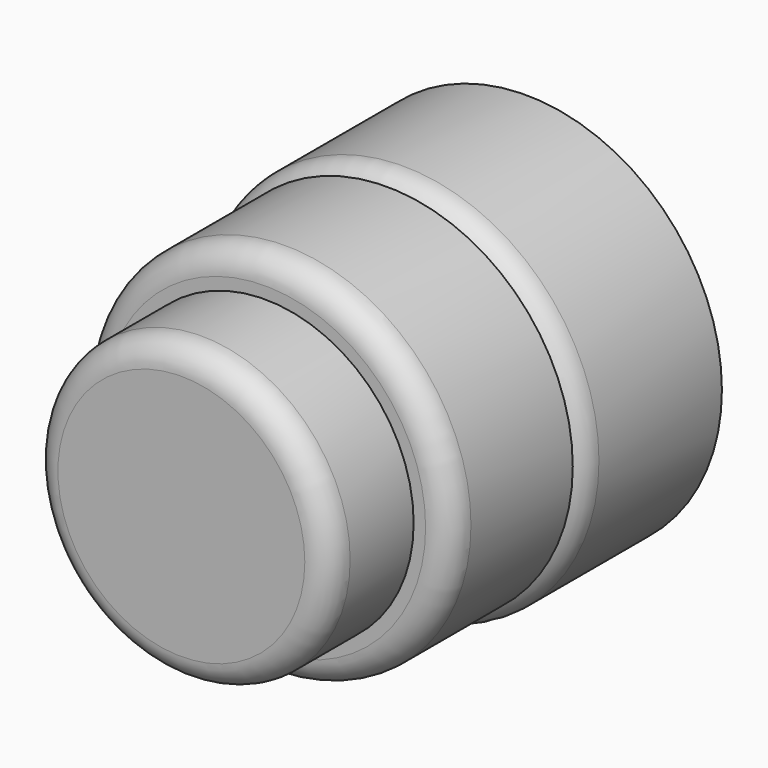
from build123d import *

# Parameters (mm, degrees)
F0_R     = 39.497
F1_DEPTH = 91.186
F2_R     = 39.497
F2_R_2   = 37.465
F3_DEPTH = 56.134
F4_R     = 37.465
F4_R_2   = 32.893
F5_DEPTH = 25.4
F6_R     = 29.972
F7_DEPTH = 21.082
F9_DEPTH = 17.78


# Not quite as in the source:
# - a fillet or chamfer that OpenCascade refuses, or shapes differently, is made with other operations: its cross-section is extruded or revolved along the edge and cut away or added


with BuildPart() as f1:
    # F0 (on Front) → F1 (new body)
    with BuildSketch(Plane.XZ):
        Circle(F0_R)
    extrude(amount=F1_DEPTH)

    # F2 (on face) → F3 (cut)
    with BuildSketch(Plane.XZ.offset(91.186)):
        Circle(F2_R)
        Circle(F2_R_2, mode=Mode.SUBTRACT)
    extrude(amount=-F3_DEPTH, mode=Mode.SUBTRACT)

    # F4 (on face) → F5 (cut)
    with BuildSketch(Plane.XZ.offset(91.186)):
        Circle(F4_R)
        Circle(F4_R_2, mode=Mode.SUBTRACT)
        Circle(F4_R_2)
    extrude(amount=-F5_DEPTH, mode=Mode.SUBTRACT)

    # F6 (on face) → F7 (join)
    with BuildSketch(Plane.XZ.offset(65.786)):
        Circle(F6_R)
    extrude(amount=F7_DEPTH)

    # F8 (on face) → F9 (cut)
    with BuildSketch(Plane(origin=(0, 0, 0), x_dir=(-1, 0, 0), z_dir=(0, 1, 0))):
        with BuildLine():
            ThreePointArc((0, 23.3172), (1.113551759, 23.778448241), (1.5748, 24.892))
            ThreePointArc((1.5748, 24.892), (1.113551759, 26.005551759), (0, 26.4668))
            ThreePointArc((0, 26.4668), (-1.5748, 24.892), (0, 23.3172))
        make_face()
        with BuildLine():
            ThreePointArc((26.4668, 0), (24.892, 1.5748), (23.3172, 0))
            ThreePointArc((23.3172, 0), (24.892, -1.5748), (26.4668, 0))
        make_face()
        with BuildLine():
            ThreePointArc((1.5748, -24.892), (1.113551759, -23.778448241), (0, -23.3172))
            ThreePointArc((0, -23.3172), (-1.5748, -24.892), (0, -26.4668))
            ThreePointArc((0, -26.4668), (1.113551759, -26.005551759), (1.5748, -24.892))
        make_face()
        with BuildLine():
            ThreePointArc((-26.4668, 0), (-24.892, -1.5748), (-23.3172, 0))
            ThreePointArc((-23.3172, 0), (-24.892, 1.5748), (-26.4668, 0))
        make_face()
    extrude(amount=-F9_DEPTH, mode=Mode.SUBTRACT)

    # F10: fillet of radius 5.08 on 3 edges, made by hand

    # F10_s1 → F10_t2 (revolve, cut)
    with BuildSketch(Plane.XY):
        with BuildLine():
            ThreePointArc((37.465, -60.706), (35.9771024484, -64.2981024484), (32.385, -65.786))
            Line((32.385, -65.786), (37.465, -65.786))
            Line((37.465, -65.786), (37.465, -60.706))
        make_face()
    revolve(axis=Axis((0, -65.786, 0), (0, -1, 0)), mode=Mode.SUBTRACT)

    # F10_s3 → F10_t4 (revolve, cut)
    with BuildSketch(Plane.XY):
        with BuildLine():
            ThreePointArc((39.497, -30.988), (38.9606901303, -33.2598450651), (37.465, -35.052))
            Line((37.465, -35.052), (39.497, -35.052))
            Line((39.497, -35.052), (39.497, -30.988))
        make_face()
    revolve(axis=Axis((0, -35.052, 0), (0, -1, 0)), mode=Mode.SUBTRACT)

    # F10_s5 → F10_t6 (revolve, cut)
    with BuildSketch(Plane.XY):
        with BuildLine():
            ThreePointArc((29.972, -81.788), (28.4841024484, -85.3801024484), (24.892, -86.868))
            Line((24.892, -86.868), (29.972, -86.868))
            Line((29.972, -86.868), (29.972, -81.788))
        make_face()
    revolve(axis=Axis((0, -86.868, 0), (0, -1, 0)), mode=Mode.SUBTRACT)


solid = f1.part
